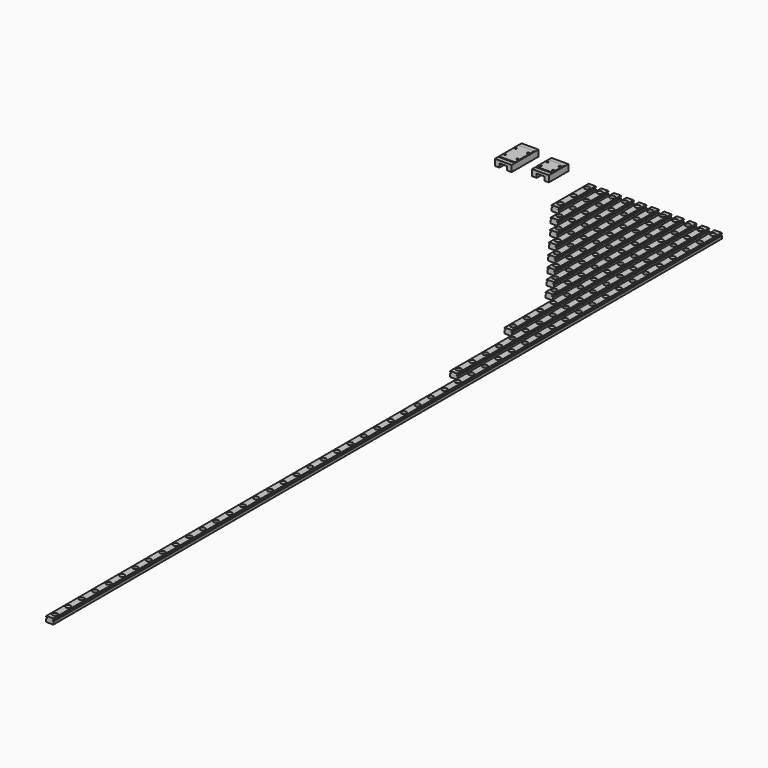
from build123d import *

# Parameters (mm, degrees)
F1_DEPTH           = 55
F2_DEPTH           = 75
F3_DEPTH           = 95
F4_DEPTH           = 115
F5_DEPTH           = 135
F6_DEPTH           = 155
F7_DEPTH           = 175
F8_DEPTH           = 195
F9_DEPTH           = 275
F10_DEPTH          = 375
F11_DEPTH          = 995
F13_D              = 3.5
F13_CBORE_D        = 6
F13_CBORE_DEPTH    = 3.5
F13_2_D            = 3.5
F13_2_CBORE_D      = 6
F13_2_CBORE_DEPTH  = 3.5
F13_3_D            = 3.5
F13_3_CBORE_D      = 6
F13_3_CBORE_DEPTH  = 3.5
F13_4_D            = 3.5
F13_4_CBORE_D      = 6
F13_4_CBORE_DEPTH  = 3.5
F13_5_D            = 3.5
F13_5_CBORE_D      = 6
F13_5_CBORE_DEPTH  = 3.5
F13_6_D            = 3.5
F13_6_CBORE_D      = 6
F13_6_CBORE_DEPTH  = 3.5
F13_7_D            = 3.5
F13_7_CBORE_D      = 6
F13_7_CBORE_DEPTH  = 3.5
F13_8_D            = 3.5
F13_8_CBORE_D      = 6
F13_8_CBORE_DEPTH  = 3.5
F13_9_D            = 3.5
F13_9_CBORE_D      = 6
F13_9_CBORE_DEPTH  = 3.5
F13_10_D           = 3.5
F13_10_CBORE_D     = 6
F13_10_CBORE_DEPTH = 3.5
F14_D              = 3.5
F14_CBORE_D        = 6
F14_CBORE_DEPTH    = 3.5
F16_DEPTH          = 9.45
F18_DEPTH          = 5
F19_DEPTH          = 14.95
F21_DEPTH          = 5
F23_D              = 2.5
F23_DEPTH          = 4.1
F23_TIP            = 0.7510757738
F23_2_D            = 2.5
F23_2_DEPTH        = 4.1
F23_2_TIP          = 0.7510757738
F25_SIZE           = 0.49999


# Not quite as in the source:
# - a fillet or chamfer is up to 0.001 mm smaller than in the source, because OpenCascade refuses the exact size


with BuildPart() as f1:
    # F0 (on Front) → F1 (new body)
    with BuildSketch(Plane.XZ):
        with BuildLine():
            Line((-4.1464466094, -3.25), (4.1464466094, -3.25))
            Line((4.1464466094, -3.25), (4.5, -2.8964466094))
            Line((4.5, -2.8964466094), (4.5, 0.2817541634))
            ThreePointArc((4.5, 0.2817541634), (4.1012202029, 0.4890238013), (3.833484861, 0.85))
            Line((3.833484861, 0.85), (3.3, 0.85))
            Line((3.3, 0.85), (3.3, 1.65))
            Line((3.3, 1.65), (3.833484861, 1.65))
            ThreePointArc((3.833484861, 1.65), (4.1012202029, 2.0109761987), (4.5, 2.2182458366))
            Line((4.5, 2.2182458366), (4.5, 2.8964466094))
            Line((4.5, 2.8964466094), (4.1464466094, 3.25))
            Line((4.1464466094, 3.25), (-4.1464466094, 3.25))
            Line((-4.1464466094, 3.25), (-4.5, 2.8964466094))
            Line((-4.5, 2.8964466094), (-4.5, 2.2182458366))
            ThreePointArc((-4.5, 2.2182458366), (-4.1012202029, 2.0109761987), (-3.833484861, 1.65))
            Line((-3.833484861, 1.65), (-3.3, 1.65))
            Line((-3.3, 1.65), (-3.3, 0.85))
            Line((-3.3, 0.85), (-3.833484861, 0.85))
            ThreePointArc((-3.833484861, 0.85), (-4.1012202029, 0.4890238013), (-4.5, 0.2817541634))
            Line((-4.5, 0.2817541634), (-4.5, -2.8964466094))
            Line((-4.5, -2.8964466094), (-4.1464466094, -3.25))
        make_face()
    extrude(amount=F1_DEPTH)

    # F13 (through all)
    with Locations(Plane.XY.offset(3.25)):
        with Locations((75, -7.5), (135, -47.5), (15, -47.5), (60, -7.5), (90, -27.5), (90, -47.5), (120, -27.5), (30, -7.5), (105, -7.5), (30, -47.5), (0, -47.5), (75, -47.5), (45, -7.5), (90, -7.5), (120, -47.5), (105, -27.5), (15, -7.5), (105, -47.5), (75, -27.5), (135, -27.5), (45, -47.5), (0, -7.5), (60, -47.5), (30, -27.5), (120, -7.5), (45, -27.5), (135, -7.5), (60, -27.5), (0, -27.5), (15, -27.5), (135, -67.5), (30, -67.5), (120, -67.5), (45, -67.5), (15, -67.5), (105, -67.5), (60, -67.5), (75, -67.5), (90, -67.5), (30, -87.5), (45, -87.5), (75, -87.5), (60, -87.5), (105, -87.5), (90, -87.5), (135, -87.5), (120, -87.5), (75, -107.5), (45, -107.5), (60, -107.5), (135, -107.5), (105, -107.5), (120, -107.5), (90, -107.5), (135, -127.5), (105, -127.5), (120, -127.5), (60, -127.5), (75, -127.5), (90, -127.5), (75, -147.5), (90, -147.5), (120, -147.5), (105, -147.5), (135, -147.5), (90, -167.5), (105, -167.5), (135, -167.5), (120, -167.5), (135, -187.5), (105, -187.5), (120, -187.5), (120, -227.5), (135, -267.5), (135, -227.5), (120, -267.5), (120, -207.5), (135, -207.5), (135, -247.5), (120, -247.5), (135, -307.5), (135, -347.5), (135, -367.5), (135, -327.5), (135, -287.5)):
            CounterBoreHole(F13_D / 2, F13_CBORE_D / 2, F13_CBORE_DEPTH)


with BuildPart() as f2:
    # F0 (on Front) → F2 (new body)
    with BuildSketch(Plane.XZ):
        with BuildLine():
            Line((10.5, 0.2817541634), (10.5, -2.8964466094))
            Line((10.5, -2.8964466094), (10.8535533906, -3.25))
            Line((10.8535533906, -3.25), (19.1464466094, -3.25))
            Line((19.1464466094, -3.25), (19.5, -2.8964466094))
            Line((19.5, -2.8964466094), (19.5, 0.2817541634))
            ThreePointArc((19.5, 0.2817541634), (19.1012202029, 0.4890238013), (18.833484861, 0.85))
            Line((18.833484861, 0.85), (18.3, 0.85))
            Line((18.3, 0.85), (18.3, 1.65))
            Line((18.3, 1.65), (18.833484861, 1.65))
            ThreePointArc((18.833484861, 1.65), (19.1012202029, 2.0109761987), (19.5, 2.2182458366))
            Line((19.5, 2.2182458366), (19.5, 2.8964466094))
            Line((19.5, 2.8964466094), (19.1464466094, 3.25))
            Line((19.1464466094, 3.25), (10.8535533906, 3.25))
            Line((10.8535533906, 3.25), (10.5, 2.8964466094))
            Line((10.5, 2.8964466094), (10.5, 2.2182458366))
            ThreePointArc((10.5, 2.2182458366), (10.8987797971, 2.0109761987), (11.166515139, 1.65))
            Line((11.166515139, 1.65), (11.7, 1.65))
            Line((11.7, 1.65), (11.7, 0.85))
            Line((11.7, 0.85), (11.166515139, 0.85))
            ThreePointArc((11.166515139, 0.85), (10.8987797971, 0.4890238013), (10.5, 0.2817541634))
        make_face()
    extrude(amount=F2_DEPTH)

    # F13#2 (through all)
    with Locations(Plane.XY.offset(3.25)):
        with Locations((75, -7.5), (135, -47.5), (15, -47.5), (60, -7.5), (90, -27.5), (90, -47.5), (120, -27.5), (30, -7.5), (105, -7.5), (30, -47.5), (0, -47.5), (75, -47.5), (45, -7.5), (90, -7.5), (120, -47.5), (105, -27.5), (15, -7.5), (105, -47.5), (75, -27.5), (135, -27.5), (45, -47.5), (0, -7.5), (60, -47.5), (30, -27.5), (120, -7.5), (45, -27.5), (135, -7.5), (60, -27.5), (0, -27.5), (15, -27.5), (135, -67.5), (30, -67.5), (120, -67.5), (45, -67.5), (15, -67.5), (105, -67.5), (60, -67.5), (75, -67.5), (90, -67.5), (30, -87.5), (45, -87.5), (75, -87.5), (60, -87.5), (105, -87.5), (90, -87.5), (135, -87.5), (120, -87.5), (75, -107.5), (45, -107.5), (60, -107.5), (135, -107.5), (105, -107.5), (120, -107.5), (90, -107.5), (135, -127.5), (105, -127.5), (120, -127.5), (60, -127.5), (75, -127.5), (90, -127.5), (75, -147.5), (90, -147.5), (120, -147.5), (105, -147.5), (135, -147.5), (90, -167.5), (105, -167.5), (135, -167.5), (120, -167.5), (135, -187.5), (105, -187.5), (120, -187.5), (120, -227.5), (135, -267.5), (135, -227.5), (120, -267.5), (120, -207.5), (135, -207.5), (135, -247.5), (120, -247.5), (135, -307.5), (135, -347.5), (135, -367.5), (135, -327.5), (135, -287.5)):
            CounterBoreHole(F13_2_D / 2, F13_2_CBORE_D / 2, F13_2_CBORE_DEPTH)


with BuildPart() as f3:
    # F0 (on Front) → F3 (new body)
    with BuildSketch(Plane.XZ):
        with BuildLine():
            Line((25.5, 0.2817541634), (25.5, -2.8964466094))
            Line((25.5, -2.8964466094), (25.8535533906, -3.25))
            Line((25.8535533906, -3.25), (34.1464466094, -3.25))
            Line((34.1464466094, -3.25), (34.5, -2.8964466094))
            Line((34.5, -2.8964466094), (34.5, 0.2817541634))
            ThreePointArc((34.5, 0.2817541634), (34.1012202029, 0.4890238013), (33.833484861, 0.85))
            Line((33.833484861, 0.85), (33.3, 0.85))
            Line((33.3, 0.85), (33.3, 1.65))
            Line((33.3, 1.65), (33.833484861, 1.65))
            ThreePointArc((33.833484861, 1.65), (34.1012202029, 2.0109761987), (34.5, 2.2182458366))
            Line((34.5, 2.2182458366), (34.5, 2.8964466094))
            Line((34.5, 2.8964466094), (34.1464466094, 3.25))
            Line((34.1464466094, 3.25), (25.8535533906, 3.25))
            Line((25.8535533906, 3.25), (25.5, 2.8964466094))
            Line((25.5, 2.8964466094), (25.5, 2.2182458366))
            ThreePointArc((25.5, 2.2182458366), (25.8987797971, 2.0109761987), (26.166515139, 1.65))
            Line((26.166515139, 1.65), (26.7, 1.65))
            Line((26.7, 1.65), (26.7, 0.85))
            Line((26.7, 0.85), (26.166515139, 0.85))
            ThreePointArc((26.166515139, 0.85), (25.8987797971, 0.4890238013), (25.5, 0.2817541634))
        make_face()
    extrude(amount=F3_DEPTH)

    # F13#3 (through all)
    with Locations(Plane.XY.offset(3.25)):
        with Locations((75, -7.5), (135, -47.5), (15, -47.5), (60, -7.5), (90, -27.5), (90, -47.5), (120, -27.5), (30, -7.5), (105, -7.5), (30, -47.5), (0, -47.5), (75, -47.5), (45, -7.5), (90, -7.5), (120, -47.5), (105, -27.5), (15, -7.5), (105, -47.5), (75, -27.5), (135, -27.5), (45, -47.5), (0, -7.5), (60, -47.5), (30, -27.5), (120, -7.5), (45, -27.5), (135, -7.5), (60, -27.5), (0, -27.5), (15, -27.5), (135, -67.5), (30, -67.5), (120, -67.5), (45, -67.5), (15, -67.5), (105, -67.5), (60, -67.5), (75, -67.5), (90, -67.5), (30, -87.5), (45, -87.5), (75, -87.5), (60, -87.5), (105, -87.5), (90, -87.5), (135, -87.5), (120, -87.5), (75, -107.5), (45, -107.5), (60, -107.5), (135, -107.5), (105, -107.5), (120, -107.5), (90, -107.5), (135, -127.5), (105, -127.5), (120, -127.5), (60, -127.5), (75, -127.5), (90, -127.5), (75, -147.5), (90, -147.5), (120, -147.5), (105, -147.5), (135, -147.5), (90, -167.5), (105, -167.5), (135, -167.5), (120, -167.5), (135, -187.5), (105, -187.5), (120, -187.5), (120, -227.5), (135, -267.5), (135, -227.5), (120, -267.5), (120, -207.5), (135, -207.5), (135, -247.5), (120, -247.5), (135, -307.5), (135, -347.5), (135, -367.5), (135, -327.5), (135, -287.5)):
            CounterBoreHole(F13_3_D / 2, F13_3_CBORE_D / 2, F13_3_CBORE_DEPTH)


with BuildPart() as f4:
    # F0 (on Front) → F4 (new body)
    with BuildSketch(Plane.XZ):
        with BuildLine():
            Line((40.5, 0.2817541634), (40.5, -2.8964466094))
            Line((40.5, -2.8964466094), (40.8535533906, -3.25))
            Line((40.8535533906, -3.25), (49.1464466094, -3.25))
            Line((49.1464466094, -3.25), (49.5, -2.8964466094))
            Line((49.5, -2.8964466094), (49.5, 0.2817541634))
            ThreePointArc((49.5, 0.2817541634), (49.1012202029, 0.4890238013), (48.833484861, 0.85))
            Line((48.833484861, 0.85), (48.3, 0.85))
            Line((48.3, 0.85), (48.3, 1.65))
            Line((48.3, 1.65), (48.833484861, 1.65))
            ThreePointArc((48.833484861, 1.65), (49.1012202029, 2.0109761987), (49.5, 2.2182458366))
            Line((49.5, 2.2182458366), (49.5, 2.8964466094))
            Line((49.5, 2.8964466094), (49.1464466094, 3.25))
            Line((49.1464466094, 3.25), (40.8535533906, 3.25))
            Line((40.8535533906, 3.25), (40.5, 2.8964466094))
            Line((40.5, 2.8964466094), (40.5, 2.2182458366))
            ThreePointArc((40.5, 2.2182458366), (40.8987797971, 2.0109761987), (41.166515139, 1.65))
            Line((41.166515139, 1.65), (41.7, 1.65))
            Line((41.7, 1.65), (41.7, 0.85))
            Line((41.7, 0.85), (41.166515139, 0.85))
            ThreePointArc((41.166515139, 0.85), (40.8987797971, 0.4890238013), (40.5, 0.2817541634))
        make_face()
    extrude(amount=F4_DEPTH)

    # F13#4 (through all)
    with Locations(Plane.XY.offset(3.25)):
        with Locations((75, -7.5), (135, -47.5), (15, -47.5), (60, -7.5), (90, -27.5), (90, -47.5), (120, -27.5), (30, -7.5), (105, -7.5), (30, -47.5), (0, -47.5), (75, -47.5), (45, -7.5), (90, -7.5), (120, -47.5), (105, -27.5), (15, -7.5), (105, -47.5), (75, -27.5), (135, -27.5), (45, -47.5), (0, -7.5), (60, -47.5), (30, -27.5), (120, -7.5), (45, -27.5), (135, -7.5), (60, -27.5), (0, -27.5), (15, -27.5), (135, -67.5), (30, -67.5), (120, -67.5), (45, -67.5), (15, -67.5), (105, -67.5), (60, -67.5), (75, -67.5), (90, -67.5), (30, -87.5), (45, -87.5), (75, -87.5), (60, -87.5), (105, -87.5), (90, -87.5), (135, -87.5), (120, -87.5), (75, -107.5), (45, -107.5), (60, -107.5), (135, -107.5), (105, -107.5), (120, -107.5), (90, -107.5), (135, -127.5), (105, -127.5), (120, -127.5), (60, -127.5), (75, -127.5), (90, -127.5), (75, -147.5), (90, -147.5), (120, -147.5), (105, -147.5), (135, -147.5), (90, -167.5), (105, -167.5), (135, -167.5), (120, -167.5), (135, -187.5), (105, -187.5), (120, -187.5), (120, -227.5), (135, -267.5), (135, -227.5), (120, -267.5), (120, -207.5), (135, -207.5), (135, -247.5), (120, -247.5), (135, -307.5), (135, -347.5), (135, -367.5), (135, -327.5), (135, -287.5)):
            CounterBoreHole(F13_4_D / 2, F13_4_CBORE_D / 2, F13_4_CBORE_DEPTH)


with BuildPart() as f5:
    # F0 (on Front) → F5 (new body)
    with BuildSketch(Plane.XZ):
        with BuildLine():
            Line((55.5, 0.2817541634), (55.5, -2.8964466094))
            Line((55.5, -2.8964466094), (55.8535533906, -3.25))
            Line((55.8535533906, -3.25), (64.1464466094, -3.25))
            Line((64.1464466094, -3.25), (64.5, -2.8964466094))
            Line((64.5, -2.8964466094), (64.5, 0.2817541634))
            ThreePointArc((64.5, 0.2817541634), (64.1012202029, 0.4890238013), (63.833484861, 0.85))
            Line((63.833484861, 0.85), (63.3, 0.85))
            Line((63.3, 0.85), (63.3, 1.65))
            Line((63.3, 1.65), (63.833484861, 1.65))
            ThreePointArc((63.833484861, 1.65), (64.1012202029, 2.0109761987), (64.5, 2.2182458366))
            Line((64.5, 2.2182458366), (64.5, 2.8964466094))
            Line((64.5, 2.8964466094), (64.1464466094, 3.25))
            Line((64.1464466094, 3.25), (55.8535533906, 3.25))
            Line((55.8535533906, 3.25), (55.5, 2.8964466094))
            Line((55.5, 2.8964466094), (55.5, 2.2182458366))
            ThreePointArc((55.5, 2.2182458366), (55.8987797971, 2.0109761987), (56.166515139, 1.65))
            Line((56.166515139, 1.65), (56.7, 1.65))
            Line((56.7, 1.65), (56.7, 0.85))
            Line((56.7, 0.85), (56.166515139, 0.85))
            ThreePointArc((56.166515139, 0.85), (55.8987797971, 0.4890238013), (55.5, 0.2817541634))
        make_face()
    extrude(amount=F5_DEPTH)

    # F13#5 (through all)
    with Locations(Plane.XY.offset(3.25)):
        with Locations((75, -7.5), (135, -47.5), (15, -47.5), (60, -7.5), (90, -27.5), (90, -47.5), (120, -27.5), (30, -7.5), (105, -7.5), (30, -47.5), (0, -47.5), (75, -47.5), (45, -7.5), (90, -7.5), (120, -47.5), (105, -27.5), (15, -7.5), (105, -47.5), (75, -27.5), (135, -27.5), (45, -47.5), (0, -7.5), (60, -47.5), (30, -27.5), (120, -7.5), (45, -27.5), (135, -7.5), (60, -27.5), (0, -27.5), (15, -27.5), (135, -67.5), (30, -67.5), (120, -67.5), (45, -67.5), (15, -67.5), (105, -67.5), (60, -67.5), (75, -67.5), (90, -67.5), (30, -87.5), (45, -87.5), (75, -87.5), (60, -87.5), (105, -87.5), (90, -87.5), (135, -87.5), (120, -87.5), (75, -107.5), (45, -107.5), (60, -107.5), (135, -107.5), (105, -107.5), (120, -107.5), (90, -107.5), (135, -127.5), (105, -127.5), (120, -127.5), (60, -127.5), (75, -127.5), (90, -127.5), (75, -147.5), (90, -147.5), (120, -147.5), (105, -147.5), (135, -147.5), (90, -167.5), (105, -167.5), (135, -167.5), (120, -167.5), (135, -187.5), (105, -187.5), (120, -187.5), (120, -227.5), (135, -267.5), (135, -227.5), (120, -267.5), (120, -207.5), (135, -207.5), (135, -247.5), (120, -247.5), (135, -307.5), (135, -347.5), (135, -367.5), (135, -327.5), (135, -287.5)):
            CounterBoreHole(F13_5_D / 2, F13_5_CBORE_D / 2, F13_5_CBORE_DEPTH)


with BuildPart() as f6:
    # F0 (on Front) → F6 (new body)
    with BuildSketch(Plane.XZ):
        with BuildLine():
            Line((70.5, 0.2817541634), (70.5, -2.8964466094))
            Line((70.5, -2.8964466094), (70.8535533906, -3.25))
            Line((70.8535533906, -3.25), (79.1464466094, -3.25))
            Line((79.1464466094, -3.25), (79.5, -2.8964466094))
            Line((79.5, -2.8964466094), (79.5, 0.2817541634))
            ThreePointArc((79.5, 0.2817541634), (79.1012202029, 0.4890238013), (78.833484861, 0.85))
            Line((78.833484861, 0.85), (78.3, 0.85))
            Line((78.3, 0.85), (78.3, 1.65))
            Line((78.3, 1.65), (78.833484861, 1.65))
            ThreePointArc((78.833484861, 1.65), (79.1012202029, 2.0109761987), (79.5, 2.2182458366))
            Line((79.5, 2.2182458366), (79.5, 2.8964466094))
            Line((79.5, 2.8964466094), (79.1464466094, 3.25))
            Line((79.1464466094, 3.25), (70.8535533906, 3.25))
            Line((70.8535533906, 3.25), (70.5, 2.8964466094))
            Line((70.5, 2.8964466094), (70.5, 2.2182458366))
            ThreePointArc((70.5, 2.2182458366), (70.8987797971, 2.0109761987), (71.166515139, 1.65))
            Line((71.166515139, 1.65), (71.7, 1.65))
            Line((71.7, 1.65), (71.7, 0.85))
            Line((71.7, 0.85), (71.166515139, 0.85))
            ThreePointArc((71.166515139, 0.85), (70.8987797971, 0.4890238013), (70.5, 0.2817541634))
        make_face()
    extrude(amount=F6_DEPTH)

    # F13#6 (through all)
    with Locations(Plane.XY.offset(3.25)):
        with Locations((75, -7.5), (135, -47.5), (15, -47.5), (60, -7.5), (90, -27.5), (90, -47.5), (120, -27.5), (30, -7.5), (105, -7.5), (30, -47.5), (0, -47.5), (75, -47.5), (45, -7.5), (90, -7.5), (120, -47.5), (105, -27.5), (15, -7.5), (105, -47.5), (75, -27.5), (135, -27.5), (45, -47.5), (0, -7.5), (60, -47.5), (30, -27.5), (120, -7.5), (45, -27.5), (135, -7.5), (60, -27.5), (0, -27.5), (15, -27.5), (135, -67.5), (30, -67.5), (120, -67.5), (45, -67.5), (15, -67.5), (105, -67.5), (60, -67.5), (75, -67.5), (90, -67.5), (30, -87.5), (45, -87.5), (75, -87.5), (60, -87.5), (105, -87.5), (90, -87.5), (135, -87.5), (120, -87.5), (75, -107.5), (45, -107.5), (60, -107.5), (135, -107.5), (105, -107.5), (120, -107.5), (90, -107.5), (135, -127.5), (105, -127.5), (120, -127.5), (60, -127.5), (75, -127.5), (90, -127.5), (75, -147.5), (90, -147.5), (120, -147.5), (105, -147.5), (135, -147.5), (90, -167.5), (105, -167.5), (135, -167.5), (120, -167.5), (135, -187.5), (105, -187.5), (120, -187.5), (120, -227.5), (135, -267.5), (135, -227.5), (120, -267.5), (120, -207.5), (135, -207.5), (135, -247.5), (120, -247.5), (135, -307.5), (135, -347.5), (135, -367.5), (135, -327.5), (135, -287.5)):
            CounterBoreHole(F13_6_D / 2, F13_6_CBORE_D / 2, F13_6_CBORE_DEPTH)


with BuildPart() as f7:
    # F0 (on Front) → F7 (new body)
    with BuildSketch(Plane.XZ):
        with BuildLine():
            Line((85.5, 0.2817541634), (85.5, -2.8964466094))
            Line((85.5, -2.8964466094), (85.8535533906, -3.25))
            Line((85.8535533906, -3.25), (94.1464466094, -3.25))
            Line((94.1464466094, -3.25), (94.5, -2.8964466094))
            Line((94.5, -2.8964466094), (94.5, 0.2817541634))
            ThreePointArc((94.5, 0.2817541634), (94.1012202029, 0.4890238013), (93.833484861, 0.85))
            Line((93.833484861, 0.85), (93.3, 0.85))
            Line((93.3, 0.85), (93.3, 1.65))
            Line((93.3, 1.65), (93.833484861, 1.65))
            ThreePointArc((93.833484861, 1.65), (94.1012202029, 2.0109761987), (94.5, 2.2182458366))
            Line((94.5, 2.2182458366), (94.5, 2.8964466094))
            Line((94.5, 2.8964466094), (94.1464466094, 3.25))
            Line((94.1464466094, 3.25), (85.8535533906, 3.25))
            Line((85.8535533906, 3.25), (85.5, 2.8964466094))
            Line((85.5, 2.8964466094), (85.5, 2.2182458366))
            ThreePointArc((85.5, 2.2182458366), (85.8987797971, 2.0109761987), (86.166515139, 1.65))
            Line((86.166515139, 1.65), (86.7, 1.65))
            Line((86.7, 1.65), (86.7, 0.85))
            Line((86.7, 0.85), (86.166515139, 0.85))
            ThreePointArc((86.166515139, 0.85), (85.8987797971, 0.4890238013), (85.5, 0.2817541634))
        make_face()
    extrude(amount=F7_DEPTH)

    # F13#7 (through all)
    with Locations(Plane.XY.offset(3.25)):
        with Locations((75, -7.5), (135, -47.5), (15, -47.5), (60, -7.5), (90, -27.5), (90, -47.5), (120, -27.5), (30, -7.5), (105, -7.5), (30, -47.5), (0, -47.5), (75, -47.5), (45, -7.5), (90, -7.5), (120, -47.5), (105, -27.5), (15, -7.5), (105, -47.5), (75, -27.5), (135, -27.5), (45, -47.5), (0, -7.5), (60, -47.5), (30, -27.5), (120, -7.5), (45, -27.5), (135, -7.5), (60, -27.5), (0, -27.5), (15, -27.5), (135, -67.5), (30, -67.5), (120, -67.5), (45, -67.5), (15, -67.5), (105, -67.5), (60, -67.5), (75, -67.5), (90, -67.5), (30, -87.5), (45, -87.5), (75, -87.5), (60, -87.5), (105, -87.5), (90, -87.5), (135, -87.5), (120, -87.5), (75, -107.5), (45, -107.5), (60, -107.5), (135, -107.5), (105, -107.5), (120, -107.5), (90, -107.5), (135, -127.5), (105, -127.5), (120, -127.5), (60, -127.5), (75, -127.5), (90, -127.5), (75, -147.5), (90, -147.5), (120, -147.5), (105, -147.5), (135, -147.5), (90, -167.5), (105, -167.5), (135, -167.5), (120, -167.5), (135, -187.5), (105, -187.5), (120, -187.5), (120, -227.5), (135, -267.5), (135, -227.5), (120, -267.5), (120, -207.5), (135, -207.5), (135, -247.5), (120, -247.5), (135, -307.5), (135, -347.5), (135, -367.5), (135, -327.5), (135, -287.5)):
            CounterBoreHole(F13_7_D / 2, F13_7_CBORE_D / 2, F13_7_CBORE_DEPTH)


with BuildPart() as f8:
    # F0 (on Front) → F8 (new body)
    with BuildSketch(Plane.XZ):
        with BuildLine():
            Line((100.5, 0.2817541634), (100.5, -2.8964466094))
            Line((100.5, -2.8964466094), (100.8535533906, -3.25))
            Line((100.8535533906, -3.25), (109.1464466094, -3.25))
            Line((109.1464466094, -3.25), (109.5, -2.8964466094))
            Line((109.5, -2.8964466094), (109.5, 0.2817541634))
            ThreePointArc((109.5, 0.2817541634), (109.1012202029, 0.4890238013), (108.833484861, 0.85))
            Line((108.833484861, 0.85), (108.3, 0.85))
            Line((108.3, 0.85), (108.3, 1.65))
            Line((108.3, 1.65), (108.833484861, 1.65))
            ThreePointArc((108.833484861, 1.65), (109.1012202029, 2.0109761987), (109.5, 2.2182458366))
            Line((109.5, 2.2182458366), (109.5, 2.8964466094))
            Line((109.5, 2.8964466094), (109.1464466094, 3.25))
            Line((109.1464466094, 3.25), (100.8535533906, 3.25))
            Line((100.8535533906, 3.25), (100.5, 2.8964466094))
            Line((100.5, 2.8964466094), (100.5, 2.2182458366))
            ThreePointArc((100.5, 2.2182458366), (100.8987797971, 2.0109761987), (101.166515139, 1.65))
            Line((101.166515139, 1.65), (101.7, 1.65))
            Line((101.7, 1.65), (101.7, 0.85))
            Line((101.7, 0.85), (101.166515139, 0.85))
            ThreePointArc((101.166515139, 0.85), (100.8987797971, 0.4890238013), (100.5, 0.2817541634))
        make_face()
    extrude(amount=F8_DEPTH)

    # F13#8 (through all)
    with Locations(Plane.XY.offset(3.25)):
        with Locations((75, -7.5), (135, -47.5), (15, -47.5), (60, -7.5), (90, -27.5), (90, -47.5), (120, -27.5), (30, -7.5), (105, -7.5), (30, -47.5), (0, -47.5), (75, -47.5), (45, -7.5), (90, -7.5), (120, -47.5), (105, -27.5), (15, -7.5), (105, -47.5), (75, -27.5), (135, -27.5), (45, -47.5), (0, -7.5), (60, -47.5), (30, -27.5), (120, -7.5), (45, -27.5), (135, -7.5), (60, -27.5), (0, -27.5), (15, -27.5), (135, -67.5), (30, -67.5), (120, -67.5), (45, -67.5), (15, -67.5), (105, -67.5), (60, -67.5), (75, -67.5), (90, -67.5), (30, -87.5), (45, -87.5), (75, -87.5), (60, -87.5), (105, -87.5), (90, -87.5), (135, -87.5), (120, -87.5), (75, -107.5), (45, -107.5), (60, -107.5), (135, -107.5), (105, -107.5), (120, -107.5), (90, -107.5), (135, -127.5), (105, -127.5), (120, -127.5), (60, -127.5), (75, -127.5), (90, -127.5), (75, -147.5), (90, -147.5), (120, -147.5), (105, -147.5), (135, -147.5), (90, -167.5), (105, -167.5), (135, -167.5), (120, -167.5), (135, -187.5), (105, -187.5), (120, -187.5), (120, -227.5), (135, -267.5), (135, -227.5), (120, -267.5), (120, -207.5), (135, -207.5), (135, -247.5), (120, -247.5), (135, -307.5), (135, -347.5), (135, -367.5), (135, -327.5), (135, -287.5)):
            CounterBoreHole(F13_8_D / 2, F13_8_CBORE_D / 2, F13_8_CBORE_DEPTH)


with BuildPart() as f9:
    # F0 (on Front) → F9 (new body)
    with BuildSketch(Plane.XZ):
        with BuildLine():
            Line((115.5, 0.2817541634), (115.5, -2.8964466094))
            Line((115.5, -2.8964466094), (115.8535533906, -3.25))
            Line((115.8535533906, -3.25), (124.1464466094, -3.25))
            Line((124.1464466094, -3.25), (124.5, -2.8964466094))
            Line((124.5, -2.8964466094), (124.5, 0.2817541634))
            ThreePointArc((124.5, 0.2817541634), (124.1012202029, 0.4890238013), (123.833484861, 0.85))
            Line((123.833484861, 0.85), (123.3, 0.85))
            Line((123.3, 0.85), (123.3, 1.65))
            Line((123.3, 1.65), (123.833484861, 1.65))
            ThreePointArc((123.833484861, 1.65), (124.1012202029, 2.0109761987), (124.5, 2.2182458366))
            Line((124.5, 2.2182458366), (124.5, 2.8964466094))
            Line((124.5, 2.8964466094), (124.1464466094, 3.25))
            Line((124.1464466094, 3.25), (115.8535533906, 3.25))
            Line((115.8535533906, 3.25), (115.5, 2.8964466094))
            Line((115.5, 2.8964466094), (115.5, 2.2182458366))
            ThreePointArc((115.5, 2.2182458366), (115.8987797971, 2.0109761987), (116.166515139, 1.65))
            Line((116.166515139, 1.65), (116.7, 1.65))
            Line((116.7, 1.65), (116.7, 0.85))
            Line((116.7, 0.85), (116.166515139, 0.85))
            ThreePointArc((116.166515139, 0.85), (115.8987797971, 0.4890238013), (115.5, 0.2817541634))
        make_face()
    extrude(amount=F9_DEPTH)

    # F13#9 (through all)
    with Locations(Plane.XY.offset(3.25)):
        with Locations((75, -7.5), (135, -47.5), (15, -47.5), (60, -7.5), (90, -27.5), (90, -47.5), (120, -27.5), (30, -7.5), (105, -7.5), (30, -47.5), (0, -47.5), (75, -47.5), (45, -7.5), (90, -7.5), (120, -47.5), (105, -27.5), (15, -7.5), (105, -47.5), (75, -27.5), (135, -27.5), (45, -47.5), (0, -7.5), (60, -47.5), (30, -27.5), (120, -7.5), (45, -27.5), (135, -7.5), (60, -27.5), (0, -27.5), (15, -27.5), (135, -67.5), (30, -67.5), (120, -67.5), (45, -67.5), (15, -67.5), (105, -67.5), (60, -67.5), (75, -67.5), (90, -67.5), (30, -87.5), (45, -87.5), (75, -87.5), (60, -87.5), (105, -87.5), (90, -87.5), (135, -87.5), (120, -87.5), (75, -107.5), (45, -107.5), (60, -107.5), (135, -107.5), (105, -107.5), (120, -107.5), (90, -107.5), (135, -127.5), (105, -127.5), (120, -127.5), (60, -127.5), (75, -127.5), (90, -127.5), (75, -147.5), (90, -147.5), (120, -147.5), (105, -147.5), (135, -147.5), (90, -167.5), (105, -167.5), (135, -167.5), (120, -167.5), (135, -187.5), (105, -187.5), (120, -187.5), (120, -227.5), (135, -267.5), (135, -227.5), (120, -267.5), (120, -207.5), (135, -207.5), (135, -247.5), (120, -247.5), (135, -307.5), (135, -347.5), (135, -367.5), (135, -327.5), (135, -287.5)):
            CounterBoreHole(F13_9_D / 2, F13_9_CBORE_D / 2, F13_9_CBORE_DEPTH)


with BuildPart() as f10:
    # F0 (on Front) → F10 (new body)
    with BuildSketch(Plane.XZ):
        with BuildLine():
            Line((130.5, 0.2817541634), (130.5, -2.8964466094))
            Line((130.5, -2.8964466094), (130.8535533906, -3.25))
            Line((130.8535533906, -3.25), (139.1464466094, -3.25))
            Line((139.1464466094, -3.25), (139.5, -2.8964466094))
            Line((139.5, -2.8964466094), (139.5, 0.2817541634))
            ThreePointArc((139.5, 0.2817541634), (139.1012202029, 0.4890238013), (138.833484861, 0.85))
            Line((138.833484861, 0.85), (138.3, 0.85))
            Line((138.3, 0.85), (138.3, 1.65))
            Line((138.3, 1.65), (138.833484861, 1.65))
            ThreePointArc((138.833484861, 1.65), (139.1012202029, 2.0109761987), (139.5, 2.2182458366))
            Line((139.5, 2.2182458366), (139.5, 2.8964466094))
            Line((139.5, 2.8964466094), (139.1464466094, 3.25))
            Line((139.1464466094, 3.25), (130.8535533906, 3.25))
            Line((130.8535533906, 3.25), (130.5, 2.8964466094))
            Line((130.5, 2.8964466094), (130.5, 2.2182458366))
            ThreePointArc((130.5, 2.2182458366), (130.8987797971, 2.0109761987), (131.166515139, 1.65))
            Line((131.166515139, 1.65), (131.7, 1.65))
            Line((131.7, 1.65), (131.7, 0.85))
            Line((131.7, 0.85), (131.166515139, 0.85))
            ThreePointArc((131.166515139, 0.85), (130.8987797971, 0.4890238013), (130.5, 0.2817541634))
        make_face()
    extrude(amount=F10_DEPTH)

    # F13#10 (through all)
    with Locations(Plane.XY.offset(3.25)):
        with Locations((75, -7.5), (135, -47.5), (15, -47.5), (60, -7.5), (90, -27.5), (90, -47.5), (120, -27.5), (30, -7.5), (105, -7.5), (30, -47.5), (0, -47.5), (75, -47.5), (45, -7.5), (90, -7.5), (120, -47.5), (105, -27.5), (15, -7.5), (105, -47.5), (75, -27.5), (135, -27.5), (45, -47.5), (0, -7.5), (60, -47.5), (30, -27.5), (120, -7.5), (45, -27.5), (135, -7.5), (60, -27.5), (0, -27.5), (15, -27.5), (135, -67.5), (30, -67.5), (120, -67.5), (45, -67.5), (15, -67.5), (105, -67.5), (60, -67.5), (75, -67.5), (90, -67.5), (30, -87.5), (45, -87.5), (75, -87.5), (60, -87.5), (105, -87.5), (90, -87.5), (135, -87.5), (120, -87.5), (75, -107.5), (45, -107.5), (60, -107.5), (135, -107.5), (105, -107.5), (120, -107.5), (90, -107.5), (135, -127.5), (105, -127.5), (120, -127.5), (60, -127.5), (75, -127.5), (90, -127.5), (75, -147.5), (90, -147.5), (120, -147.5), (105, -147.5), (135, -147.5), (90, -167.5), (105, -167.5), (135, -167.5), (120, -167.5), (135, -187.5), (105, -187.5), (120, -187.5), (120, -227.5), (135, -267.5), (135, -227.5), (120, -267.5), (120, -207.5), (135, -207.5), (135, -247.5), (120, -247.5), (135, -307.5), (135, -347.5), (135, -367.5), (135, -327.5), (135, -287.5)):
            CounterBoreHole(F13_10_D / 2, F13_10_CBORE_D / 2, F13_10_CBORE_DEPTH)


with BuildPart() as f11:
    # F0 (on Front) → F11 (new body)
    with BuildSketch(Plane.XZ):
        with BuildLine():
            Line((145.5, 0.2817541634), (145.5, -2.8964466094))
            Line((145.5, -2.8964466094), (145.8535533906, -3.25))
            Line((145.8535533906, -3.25), (154.1464466094, -3.25))
            Line((154.1464466094, -3.25), (154.5, -2.8964466094))
            Line((154.5, -2.8964466094), (154.5, 0.2817541634))
            ThreePointArc((154.5, 0.2817541634), (154.1012202029, 0.4890238013), (153.833484861, 0.85))
            Line((153.833484861, 0.85), (153.3, 0.85))
            Line((153.3, 0.85), (153.3, 1.65))
            Line((153.3, 1.65), (153.833484861, 1.65))
            ThreePointArc((153.833484861, 1.65), (154.1012202029, 2.0109761987), (154.5, 2.2182458366))
            Line((154.5, 2.2182458366), (154.5, 2.8964466094))
            Line((154.5, 2.8964466094), (154.1464466094, 3.25))
            Line((154.1464466094, 3.25), (145.8535533906, 3.25))
            Line((145.8535533906, 3.25), (145.5, 2.8964466094))
            Line((145.5, 2.8964466094), (145.5, 2.2182458366))
            ThreePointArc((145.5, 2.2182458366), (145.8987797971, 2.0109761987), (146.166515139, 1.65))
            Line((146.166515139, 1.65), (146.7, 1.65))
            Line((146.7, 1.65), (146.7, 0.85))
            Line((146.7, 0.85), (146.166515139, 0.85))
            ThreePointArc((146.166515139, 0.85), (145.8987797971, 0.4890238013), (145.5, 0.2817541634))
        make_face()
    extrude(amount=F11_DEPTH)

    # F14 (through all)
    with Locations(Plane.XY.offset(3.25)):
        with Locations((150, -7.5), (150, -487.5), (150, -247.5), (150, -327.5), (150, -667.5), (150, -647.5), (150, -727.5), (150, -567.5), (150, -747.5), (150, -87.5), (150, -167.5), (150, -407.5), (150, -107.5), (150, -27.5), (150, -427.5), (150, -347.5), (150, -267.5), (150, -187.5), (150, -587.5), (150, -507.5), (150, -127.5), (150, -47.5), (150, -447.5), (150, -367.5), (150, -287.5), (150, -207.5), (150, -607.5), (150, -527.5), (150, -767.5), (150, -687.5), (150, -307.5), (150, -227.5), (150, -147.5), (150, -67.5), (150, -627.5), (150, -547.5), (150, -467.5), (150, -387.5), (150, -787.5), (150, -707.5), (150, -847.5), (150, -867.5), (150, -967.5), (150, -887.5), (150, -827.5), (150, -987.5), (150, -907.5), (150, -927.5), (150, -947.5), (150, -807.5)):
            CounterBoreHole(F14_D / 2, F14_CBORE_D / 2, F14_CBORE_DEPTH)


with BuildPart() as f16:
    # F15 (on Front) → F16 (new body)
    with BuildSketch(Plane.XZ):
        with BuildLine():
            Line((-40, 6.25), (-60, 6.25))
            Line((-60, 6.25), (-60, -1.25))
            Line((-60, -1.25), (-54.5, -1.25))
            Line((-54.5, -1.25), (-54.5, 0.25))
            ThreePointArc((-54.5, 0.25), (-55.5, 1.25), (-54.5, 2.25))
            Line((-54.5, 2.25), (-54.5, 3.25))
            Line((-54.5, 3.25), (-50, 3.25))
            Line((-50, 3.25), (-45.5, 3.25))
            Line((-45.5, 3.25), (-45.5, 2.25))
            ThreePointArc((-45.5, 2.25), (-44.5, 1.25), (-45.5, 0.25))
            Line((-45.5, 0.25), (-45.5, -1.25))
            Line((-45.5, -1.25), (-40, -1.25))
            Line((-40, -1.25), (-40, 6.25))
        make_face()
        Polygon((-40, 6.75), (-50, 6.75), (-60, 6.75), (-60, 6.25), (-40, 6.25), align=None)
    extrude(amount=F16_DEPTH)

    # F17 (on face) → F18 (join)
    with BuildSketch(Plane.XZ.offset(9.45)):
        with BuildLine():
            ThreePointArc((-54.5, 2.25), (-55.5, 1.25), (-54.5, 0.25))
            Line((-54.5, 0.25), (-54.5, 2.25))
        make_face()
        with BuildLine():
            Line((-54.5, -1.25), (-54.5, 0.25))
            ThreePointArc((-54.5, 0.25), (-55.5, 1.25), (-54.5, 2.25))
            Line((-54.5, 2.25), (-54.5, 3.25))
            Line((-54.5, 3.25), (-45.5, 3.25))
            Line((-45.5, 3.25), (-45.5, 2.25))
            ThreePointArc((-45.5, 2.25), (-44.5, 1.25), (-45.5, 0.25))
            Line((-45.5, 0.25), (-45.5, -1.25))
            Line((-45.5, -1.25), (-40, -1.25))
            Line((-40, -1.25), (-40, 6.25))
            Line((-40, 6.25), (-60, 6.25))
            Line((-60, 6.25), (-60, -1.25))
            Line((-60, -1.25), (-54.5, -1.25))
        make_face()
        with BuildLine():
            ThreePointArc((-45.5, 0.25), (-44.5, 1.25), (-45.5, 2.25))
            Line((-45.5, 2.25), (-45.5, 0.25))
        make_face()
    extrude(amount=F18_DEPTH)

    # F23
    with Locations(Plane.XY.offset(6.75)):
        with Locations((-57.5, -5), (-42.5, -5), (-82.5, -8), (-97.5, -8)):
            Hole(F23_D / 2, depth=F23_DEPTH)
            with Locations((0, 0, -(F23_DEPTH + F23_TIP / 2))):  # 118° drill point
                Cone(0, F23_D / 2, F23_TIP, mode=Mode.SUBTRACT)



with BuildPart() as f19:
    # F15 (on Front) → F19 (new body)
    with BuildSketch(Plane.XZ):
        with BuildLine():
            Line((-80, 6.25), (-100, 6.25))
            Line((-100, 6.25), (-100, -1.25))
            Line((-100, -1.25), (-94.5, -1.25))
            Line((-94.5, -1.25), (-94.5, 0.25))
            ThreePointArc((-94.5, 0.25), (-95.5, 1.25), (-94.5, 2.25))
            Line((-94.5, 2.25), (-94.5, 3.25))
            Line((-94.5, 3.25), (-90, 3.25))
            Line((-90, 3.25), (-85.5, 3.25))
            Line((-85.5, 3.25), (-85.5, 2.25))
            ThreePointArc((-85.5, 2.25), (-84.5, 1.25), (-85.5, 0.25))
            Line((-85.5, 0.25), (-85.5, -1.25))
            Line((-85.5, -1.25), (-80, -1.25))
            Line((-80, -1.25), (-80, 6.25))
        make_face()
        Polygon((-90, 6.75), (-100, 6.75), (-100, 6.25), (-80, 6.25), (-80, 6.75), align=None)
    extrude(amount=F19_DEPTH)

    # F20 (on face) → F21 (join)
    with BuildSketch(Plane.XZ.offset(14.95)):
        with BuildLine():
            Line((-94.5, -1.25), (-94.5, 0.25))
            ThreePointArc((-94.5, 0.25), (-95.5, 1.25), (-94.5, 2.25))
            Line((-94.5, 2.25), (-94.5, 3.25))
            Line((-94.5, 3.25), (-85.5, 3.25))
            Line((-85.5, 3.25), (-85.5, 2.25))
            ThreePointArc((-85.5, 2.25), (-84.5, 1.25), (-85.5, 0.25))
            Line((-85.5, 0.25), (-85.5, -1.25))
            Line((-85.5, -1.25), (-80, -1.25))
            Line((-80, -1.25), (-80, 6.25))
            Line((-80, 6.25), (-100, 6.25))
            Line((-100, 6.25), (-100, -1.25))
            Line((-100, -1.25), (-94.5, -1.25))
        make_face()
        with BuildLine():
            ThreePointArc((-94.5, 2.25), (-95.5, 1.25), (-94.5, 0.25))
            Line((-94.5, 0.25), (-94.5, 2.25))
        make_face()
        with BuildLine():
            ThreePointArc((-85.5, 0.25), (-84.5, 1.25), (-85.5, 2.25))
            Line((-85.5, 2.25), (-85.5, 0.25))
        make_face()
    extrude(amount=F21_DEPTH)

    # F23#2
    with Locations(Plane.XY.offset(6.75)):
        with Locations((-57.5, -5), (-42.5, -5), (-82.5, -8), (-97.5, -8)):
            Hole(F23_2_D / 2, depth=F23_2_DEPTH)
            with Locations((0, 0, -(F23_2_DEPTH + F23_2_TIP / 2))):  # 118° drill point
                Cone(0, F23_2_D / 2, F23_2_TIP, mode=Mode.SUBTRACT)


with BuildPart() as f16_1:
    add(f16.part)

    add(f19.part)  # F24 merges F19
    # F24: F19, F16 across face
    add(f19.part.mirror(Plane.XZ))
    add(f16.part.mirror(Plane.XZ))

    # F25 (size 0.5 in the source; OpenCascade refuses exactly that, so slightly less here)
    f25_edges = [f16_1.edges().sort_by_distance(p)[0] for p in [
        (-50, -9.45, 6.75),
        (-50, 9.45, 6.75),
        (-40, 0, 6.75),
        (-60, 0, 6.75),
        (-80, 0, 6.75),
        (-90, -14.95, 6.75),
        (-90, 14.95, 6.75),
        (-100, 0, 6.75),
    ]]
    chamfer(f25_edges, length=F25_SIZE)


solid = Compound([f1.part, f2.part, f3.part, f4.part, f5.part, f6.part, f7.part, f8.part, f9.part, f10.part, f11.part, f16_1.part])
